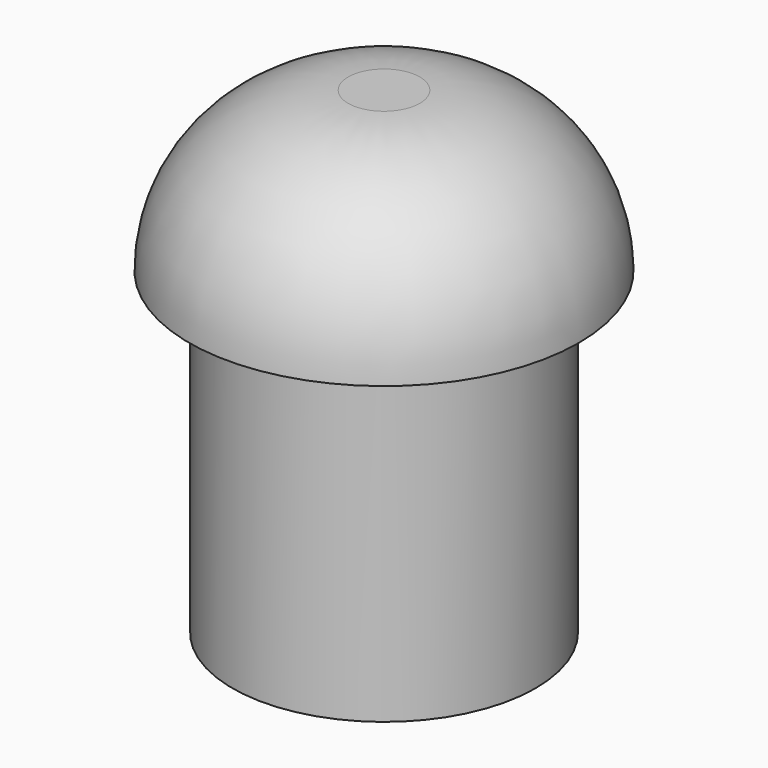
from build123d import *

# Parameters (mm, degrees)
F0_R     = 12.25
F1_DEPTH = 30
F2_R     = 12.25
F2_R_2   = 9.525
F3_DEPTH = 10
F4_DEPTH = 10
F5_R     = 9.99999


# Not quite as in the source:
# - a fillet or chamfer is up to 0.001 mm smaller than in the source, because OpenCascade refuses the exact size


with BuildPart() as f1:
    # F0 (on Top) → F1 (new body)
    with BuildSketch(Plane.XY):
        Circle(F0_R)
    extrude(amount=F1_DEPTH)

    # F2 (on face) → F3 (cut)
    with BuildSketch(Plane(origin=(0, 0, 0), x_dir=(1, 0, 0), z_dir=(0, 0, -1))):
        Circle(F2_R)
        Circle(F2_R_2, mode=Mode.SUBTRACT)
    extrude(amount=-F3_DEPTH, mode=Mode.SUBTRACT)

    # F4 (cut): a face of the model
    f4_faces = [f1.faces().sort_by_distance(p)[0] for p in [
        (-11.9035176772, 0, 10),
    ]]
    extrude(f4_faces, amount=-F4_DEPTH, mode=Mode.SUBTRACT)

    # F5 (radius 10 in the source; OpenCascade refuses exactly that, so slightly less here)
    f5_edges = [f1.edges().sort_by_distance(p)[0] for p in [
        (-12.25, 0, 30),
    ]]
    fillet(f5_edges, radius=F5_R)


solid = f1.part
